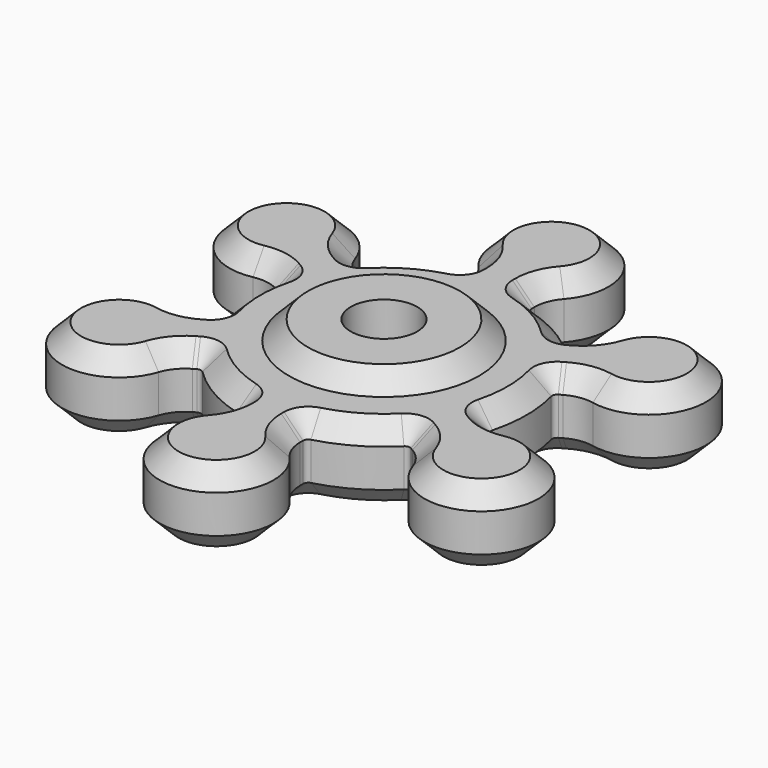
from build123d import *

# Parameters (mm, degrees)
F1_DEPTH = 4
F3_DEPTH = 2.5
F4_R     = 4
F5_DEPTH = 1
F6_R     = 1.75
F7_DEPTH = 5.001
F8_SIZE  = 0.99999


# Not quite as in the source:
# - a fillet or chamfer is up to 0.001 mm smaller than in the source, because OpenCascade refuses the exact size


with BuildPart() as f1:
    # F0 (on Top) → F1 (new body)
    with BuildSketch(Plane.XY):
        with BuildLine():
            ThreePointArc((-1.75, 7.5042031676), (-1.8060506469, 7.3388969595), (-1.9510840407, 7.2417726467))
            ThreePointArc((-1.9510840407, 7.2417726467), (-3.75, 6.4951905284), (-5.2960170601, 5.3105746675))
            ThreePointArc((-5.2960170601, 5.3105746675), (-5.4526458792, 5.2335342205), (-5.6238305783, 5.2676460404))
            Line((-5.6238305783, 5.2676460404), (-5.7871696323, 5.3619498872))
            ThreePointArc((-5.7871696323, 5.3619498872), (-6.3349564147, 5.8273689108), (-6.682813556, 6.4564004169))
            ThreePointArc((-6.682813556, 6.4564004169), (-12.124355653, 7), (-8.932813556, 2.5592860998))
            ThreePointArc((-8.932813556, 2.5592860998), (-8.2141277213, 2.5725487316), (-7.5371696323, 2.330860974))
            Line((-7.5371696323, 2.330860974), (-7.3738305783, 2.2365571272))
            ThreePointArc((-7.3738305783, 2.2365571272), (-7.2586965261, 2.105362739), (-7.2471011008, 1.9311979792))
            ThreePointArc((-7.2471011008, 1.9311979792), (-7.5, 0), (-7.2471011008, -1.9311979792))
            ThreePointArc((-7.2471011008, -1.9311979792), (-7.2586965261, -2.105362739), (-7.3738305783, -2.2365571272))
            Line((-7.3738305783, -2.2365571272), (-7.5371696323, -2.330860974))
            ThreePointArc((-7.5371696323, -2.330860974), (-8.2141277213, -2.5725487316), (-8.932813556, -2.5592860998))
            ThreePointArc((-8.932813556, -2.5592860998), (-12.124355653, -7), (-6.682813556, -6.4564004169))
            ThreePointArc((-6.682813556, -6.4564004169), (-6.3349564147, -5.8273689108), (-5.7871696323, -5.3619498872))
            Line((-5.7871696323, -5.3619498872), (-5.6238305783, -5.2676460404))
            ThreePointArc((-5.6238305783, -5.2676460404), (-5.4526458792, -5.2335342205), (-5.2960170601, -5.3105746675))
            ThreePointArc((-5.2960170601, -5.3105746675), (-3.75, -6.4951905284), (-1.9510840407, -7.2417726467))
            ThreePointArc((-1.9510840407, -7.2417726467), (-1.8060506469, -7.3388969595), (-1.75, -7.5042031676))
            Line((-1.75, -7.5042031676), (-1.75, -7.6928108612))
            ThreePointArc((-1.75, -7.6928108612), (-1.8791713066, -8.3999176424), (-2.25, -9.0156865167))
            ThreePointArc((-2.25, -9.0156865167), (0, -14), (2.25, -9.0156865167))
            ThreePointArc((2.25, -9.0156865167), (1.8791713066, -8.3999176424), (1.75, -7.6928108612))
            Line((1.75, -7.6928108612), (1.75, -7.5042031676))
            ThreePointArc((1.75, -7.5042031676), (1.8060506469, -7.3388969595), (1.9510840407, -7.2417726467))
            ThreePointArc((1.9510840407, -7.2417726467), (3.75, -6.4951905284), (5.2960170601, -5.3105746675))
            ThreePointArc((5.2960170601, -5.3105746675), (5.4526458792, -5.2335342205), (5.6238305783, -5.2676460404))
            Line((5.6238305783, -5.2676460404), (5.7871696323, -5.3619498872))
            ThreePointArc((5.7871696323, -5.3619498872), (6.3349564147, -5.8273689108), (6.682813556, -6.4564004169))
            ThreePointArc((6.682813556, -6.4564004169), (12.124355653, -7), (8.932813556, -2.5592860998))
            ThreePointArc((8.932813556, -2.5592860998), (8.2141277213, -2.5725487316), (7.5371696323, -2.330860974))
            Line((7.5371696323, -2.330860974), (7.3738305783, -2.2365571272))
            ThreePointArc((7.3738305783, -2.2365571272), (7.2586965261, -2.105362739), (7.2471011008, -1.9311979792))
            ThreePointArc((7.2471011008, -1.9311979792), (7.5, 0), (7.2471011008, 1.9311979792))
            ThreePointArc((7.2471011008, 1.9311979792), (7.2586965261, 2.105362739), (7.3738305783, 2.2365571272))
            Line((7.3738305783, 2.2365571272), (7.5371696323, 2.330860974))
            ThreePointArc((7.5371696323, 2.330860974), (8.2141277213, 2.5725487316), (8.932813556, 2.5592860998))
            ThreePointArc((8.932813556, 2.5592860998), (12.124355653, 7), (6.682813556, 6.4564004169))
            ThreePointArc((6.682813556, 6.4564004169), (6.3349564147, 5.8273689108), (5.7871696323, 5.3619498872))
            Line((5.7871696323, 5.3619498872), (5.6238305783, 5.2676460404))
            ThreePointArc((5.6238305783, 5.2676460404), (5.4526458792, 5.2335342205), (5.2960170601, 5.3105746675))
            ThreePointArc((5.2960170601, 5.3105746675), (3.75, 6.4951905284), (1.9510840407, 7.2417726467))
            ThreePointArc((1.9510840407, 7.2417726467), (1.8060506469, 7.3388969595), (1.75, 7.5042031676))
            Line((1.75, 7.5042031676), (1.75, 7.6928108612))
            ThreePointArc((1.75, 7.6928108612), (1.8791713066, 8.3999176424), (2.25, 9.0156865167))
            ThreePointArc((2.25, 9.0156865167), (0, 14), (-2.25, 9.0156865167))
            ThreePointArc((-2.25, 9.0156865167), (-1.8791713066, 8.3999176424), (-1.75, 7.6928108612))
            Line((-1.75, 7.6928108612), (-1.75, 7.5042031676))
        make_face()
    extrude(amount=F1_DEPTH)

    # F2 (on Top) → F3 (cut)
    with BuildSketch(Plane.XY):
        Polygon((2.875, -1.6598820239), (2.875, 1.6598820239), (0, 3.3197640478), (-2.875, 1.6598820239), (-2.875, -1.6598820239), (0, -3.3197640478), align=None)
    extrude(amount=F3_DEPTH, mode=Mode.SUBTRACT)

    # F4 (on face) → F5 (join)
    with BuildSketch(Plane.XY.offset(4)):
        Circle(F4_R)
    extrude(amount=F5_DEPTH)

    # F6 (on face) → F7 (cut, through all)
    with BuildSketch(Plane.XY.offset(5)):
        Circle(F6_R)
    extrude(amount=-F7_DEPTH, mode=Mode.SUBTRACT)

    # F8 (size 1 in the source; OpenCascade refuses exactly that, so slightly less here)
    f8_edges = [f1.edges().sort_by_distance(p)[0] for p in [
        (1.75, -7.598507, 4),
        (1.879171, -8.399918, 4),
        (1.806051, -7.338897, 4),
        (0, -14, 4),
        (3.75, -6.495191, 4),
        (-1.879171, -8.399918, 4),
        (5.452646, -5.233534, 4),
        (-1.75, -7.598507, 4),
        (5.7055, -5.314798, 4),
        (-1.806051, -7.338897, 4),
        (6.334956, -5.827369, 4),
        (-3.75, -6.495191, 4),
        (12.124356, -7, 4),
        (-5.452646, -5.233534, 4),
        (8.214128, -2.572549, 4),
        (-5.7055, -5.314798, 4),
        (7.4555, -2.283709, 4),
        (-6.334956, -5.827369, 4),
        (7.258697, -2.105363, 4),
        (-12.124356, -7, 4),
        (7.5, 0, 4),
        (-8.214128, -2.572549, 4),
        (7.258697, 2.105363, 4),
        (-7.4555, -2.283709, 4),
        (7.4555, 2.283709, 4),
        (-7.258697, -2.105363, 4),
        (8.214128, 2.572549, 4),
        (-7.5, 0, 4),
        (12.124356, 7, 4),
        (-7.258697, 2.105363, 4),
        (6.334956, 5.827369, 4),
        (-7.4555, 2.283709, 4),
        (5.7055, 5.314798, 4),
        (-8.214128, 2.572549, 4),
        (5.452646, 5.233534, 4),
        (-12.124356, 7, 4),
        (3.75, 6.495191, 4),
        (-6.334956, 5.827369, 4),
        (1.806051, 7.338897, 4),
        (-5.7055, 5.314798, 4),
        (1.75, 7.598507, 4),
        (-5.452646, 5.233534, 4),
        (1.879171, 8.399918, 4),
        (-3.75, 6.495191, 4),
        (0, 14, 4),
        (-1.806051, 7.338897, 4),
        (-1.879171, 8.399918, 4),
        (-1.75, 7.598507, 4),
        (-4, 0, 4),
        (-12.124356, -7, 0),
    ]]
    chamfer(f8_edges, length=F8_SIZE)


solid = f1.part
